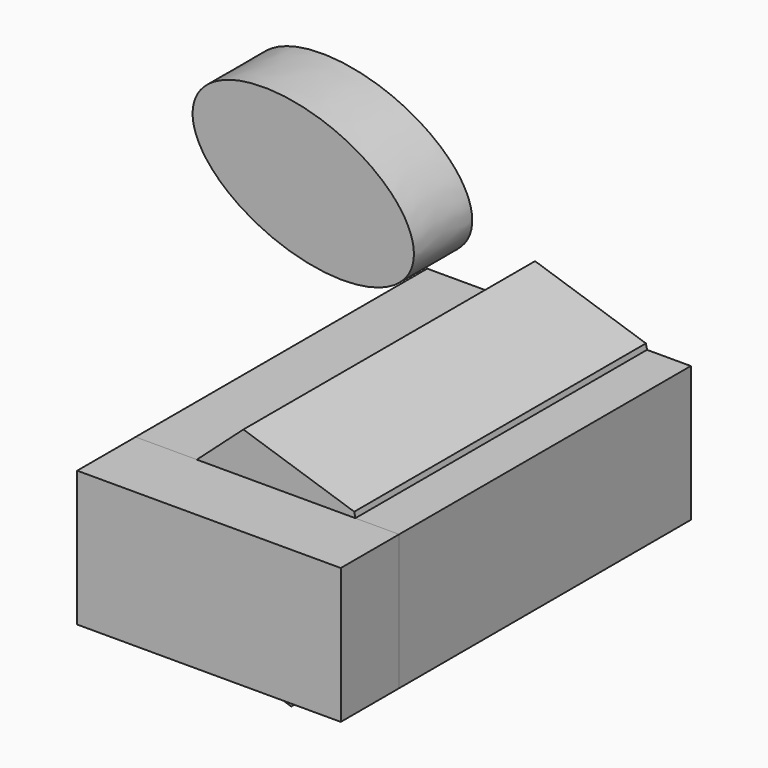
from build123d import *

# Parameters (mm, degrees)
F2_DEPTH = 125
F1_W     = 90.362906456
F1_H     = 46.4516137727
F3_DEPTH = 25
F5_DEPTH = 25


with BuildPart() as f2:
    # F0 (on Front) → F2 (new body)
    with BuildSketch(Plane.XZ):
        Polygon((-8.2146767203, 39.1474020387), (-38.0099830178, 12.4595822957), (-29.7953062975, -26.687819743), (8.2146767203, -39.1474020387), (38.0099830178, -12.4595822957), (29.7953062975, 26.687819743), align=None)
    extrude(amount=F2_DEPTH)


with BuildPart() as f2b:
    # F1 (on Front) → F2, piece 2 (new body)
    with BuildSketch(Plane.XZ):
        with Locations((0, 1.6330645885)):
            Rectangle(F1_W, F1_H)
    extrude(amount=F2_DEPTH)


with BuildPart() as f3:
    # F3 (new): a face of the model
    f3_faces = [f2b.part.faces().sort_by_distance(p)[0] for p in [
        (0, -125, 1.6330645885),
    ]]
    extrude(f3_faces, amount=F3_DEPTH)


with BuildPart() as f5:
    # F4 (on Front) → F5 (new body)
    with BuildSketch(Plane.XZ):
        with BuildLine():
            add(Edge.make_bspline(
                [(-30.4838716984, 40.1008091867), (-17.591954486, 76.3041440565), (-79.8342867277, 78.0714260498), (-142.0766189694, 79.8387080431), (-92.7262039401, 41.86809118), (-43.3757889108, 3.8974743169), (-30.4838716984, 40.1008091867)],
                knots=[0, 0, 0, 2.0943951024, 2.0943951024, 4.1887902048, 4.1887902048, 6.2831853072, 6.2831853072, 6.2831853072], degree=2, weights=[1, 0.5, 1, 0.5, 1, 0.5, 1]))
        make_face()
    extrude(amount=F5_DEPTH)


solid = Compound([f2.part, f2b.part, f3.part, f5.part])
